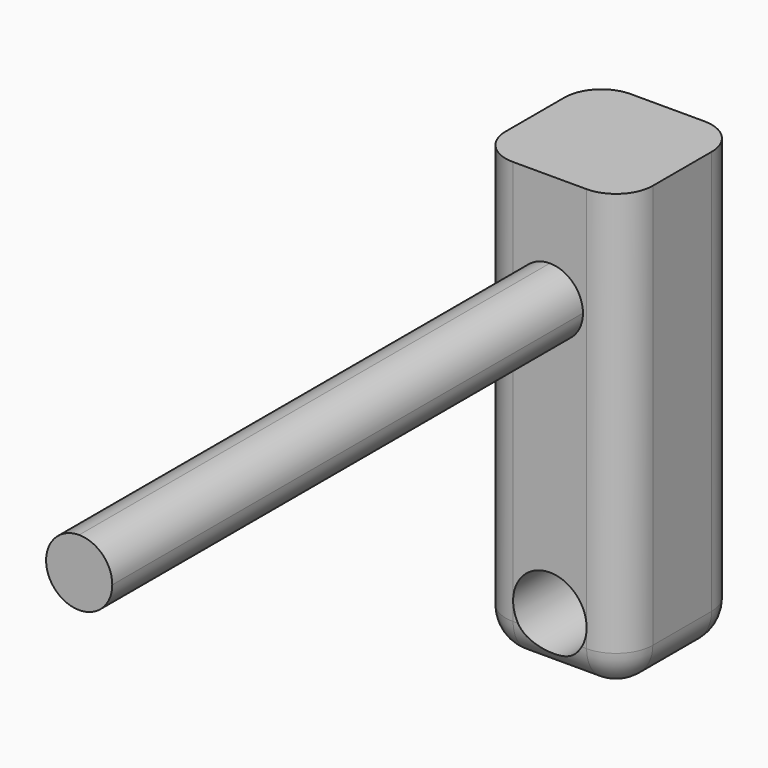
from build123d import *

# Parameters (mm, degrees)
F1_DEPTH     = 25.4
F3_DEPTH     = 101.6
F4_R         = 6.35
F6_D         = 12.7
F6_DEPTH     = 254
F6_TIP       = 3.8154649308
F7_T1_DEPTH  = 12.7
F7_T3_DEPTH  = 12.7
F7_T6_ANGLE  = 90
F7_T8_ANGLE  = 90
F7_T10_ANGLE = 90
F7_T12_ANGLE = 90


# Not quite as in the source:
# - a fillet or chamfer that OpenCascade refuses, or shapes differently, is made with other operations: its cross-section is extruded or revolved along the edge and cut away or added


with BuildPart() as f1:
    # F0 (on Front) → F1 (new body)
    with BuildSketch(Plane.XZ):
        Polygon((-12.7, -76.2), (0, -76.2), (12.7, -76.2), (12.7, 0), (-12.7, 0), align=None)
    extrude(amount=F1_DEPTH)

    # F2 (on face) → F3 (join)
    with BuildSketch(Plane.XZ.offset(25.4)):
        with BuildLine():
            ThreePointArc((5.715, -19.05), (4.0411152545, -15.0088847455), (0, -13.335))
            Line((0, -13.335), (0, -19.05))
            Line((0, -19.05), (0, -24.765))
            ThreePointArc((0, -24.765), (4.0411152545, -23.0911152545), (5.715, -19.05))
        make_face()
        with BuildLine():
            Line((0, -19.05), (0, -13.335))
            ThreePointArc((0, -13.335), (-5.715, -19.05), (0, -24.765))
            Line((0, -24.765), (0, -19.05))
        make_face()
    extrude(amount=F3_DEPTH)

    # F4
    f4_edges = [f1.edges().sort_by_distance(p)[0] for p in [
        (12.7, -25.4, -38.1),
        (12.7, 0, -38.1),
        (-12.7, -25.4, -38.1),
        (-12.7, 0, -38.1),
    ]]
    fillet(f4_edges, radius=F4_R)

    # F6
    with Locations(Plane.XZ.offset(25.4)):
        with Locations((0, -66.675)):
            Hole(F6_D / 2, depth=F6_DEPTH)
            with Locations((0, 0, -(F6_DEPTH + F6_TIP / 2))):  # 118° drill point
                Cone(0, F6_D / 2, F6_TIP, mode=Mode.SUBTRACT)

    # F7: fillet of radius 6.35 on 6 edges, made by hand

    # F7_s2 → F7_t1 (cut)
    with BuildSketch(Plane.XZ.offset(6.35)):
        with BuildLine():
            ThreePointArc((6.35, -76.2), (10.8401280605, -74.3401280605), (12.7, -69.85))
            Line((12.7, -69.85), (12.7, -76.2))
            Line((12.7, -76.2), (6.35, -76.2))
        make_face()
        with BuildLine():
            ThreePointArc((-6.35, -76.2), (-10.8401280605, -74.3401280605), (-12.7, -69.85))
            Line((-12.7, -69.85), (-12.7, -76.2))
            Line((-12.7, -76.2), (-6.35, -76.2))
        make_face()
    extrude(amount=F7_T1_DEPTH, mode=Mode.SUBTRACT)

    # F7_s4 → F7_t3 (cut)
    with BuildSketch(Plane.YZ.offset(-6.35)):
        with BuildLine():
            ThreePointArc((-19.05, -76.2), (-23.5401280605, -74.3401280605), (-25.4, -69.85))
            Line((-25.4, -69.85), (-25.4, -76.2))
            Line((-25.4, -76.2), (-19.05, -76.2))
        make_face()
        with BuildLine():
            ThreePointArc((-6.35, -76.2), (-1.8598719395, -74.3401280605), (0, -69.85))
            Line((0, -69.85), (0, -76.2))
            Line((0, -76.2), (-6.35, -76.2))
        make_face()
    extrude(amount=F7_T3_DEPTH, mode=Mode.SUBTRACT)

    # F7_s5 → F7_t6 (revolve, cut)
    with BuildSketch(Plane.XZ.offset(6.35)):
        with BuildLine():
            ThreePointArc((-6.35, -76.2), (-10.8401280605, -74.3401280605), (-12.7, -69.85))
            Line((-12.7, -69.85), (-12.7, -76.2))
            Line((-12.7, -76.2), (-6.35, -76.2))
        make_face()
    revolve(axis=Axis((-6.35, -6.35, -76.2), (0, 0, -1)), revolution_arc=F7_T6_ANGLE, mode=Mode.SUBTRACT)

    # F7_s7 → F7_t8 (revolve, cut)
    with BuildSketch(Plane.XZ.offset(19.05)):
        with BuildLine():
            ThreePointArc((-6.35, -76.2), (-10.8401280605, -74.3401280605), (-12.7, -69.85))
            Line((-12.7, -69.85), (-12.7, -76.2))
            Line((-12.7, -76.2), (-6.35, -76.2))
        make_face()
    revolve(axis=Axis((-6.35, -19.05, -76.2), (0, 0, 1)), revolution_arc=F7_T8_ANGLE, mode=Mode.SUBTRACT)

    # F7_s9 → F7_t10 (revolve, cut)
    with BuildSketch(Plane.XZ.offset(6.35)):
        with BuildLine():
            ThreePointArc((6.35, -76.2), (10.8401280605, -74.3401280605), (12.7, -69.85))
            Line((12.7, -69.85), (12.7, -76.2))
            Line((12.7, -76.2), (6.35, -76.2))
        make_face()
    revolve(axis=Axis((6.35, -6.35, -76.2), (0, 0, 1)), revolution_arc=F7_T10_ANGLE, mode=Mode.SUBTRACT)

    # F7_s11 → F7_t12 (revolve, cut)
    with BuildSketch(Plane.YZ.offset(6.35)):
        with BuildLine():
            ThreePointArc((-19.05, -76.2), (-23.5401280605, -74.3401280605), (-25.4, -69.85))
            Line((-25.4, -69.85), (-25.4, -76.2))
            Line((-25.4, -76.2), (-19.05, -76.2))
        make_face()
    revolve(axis=Axis((6.35, -19.05, -76.2), (0, 0, 1)), revolution_arc=F7_T12_ANGLE, mode=Mode.SUBTRACT)


solid = f1.part
